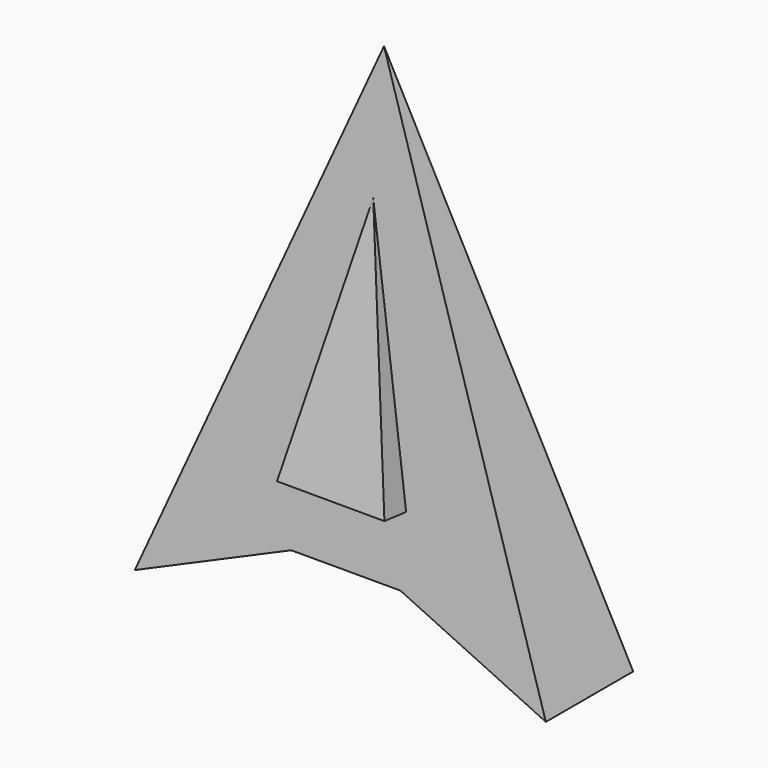
from build123d import *

# Parameters (mm, degrees)
F3_DEPTH  = 12.7
F5_DEPTH  = 67.0368353671
F6_DEPTH  = 28.5643014728
F8_DEPTH  = 6.35
F10_DEPTH = 64.56300866
F12_DEPTH = 6.35
F14_DEPTH = 65.6539037047


# Not quite as in the source:
# - the program builds the solid bodies; features that only make, move or delete a surface that nothing else refers to are left out


with BuildPart() as f3:
    # F2 (on Front) → F3 (new body, symmetric)
    with BuildSketch(Plane.XZ):
        Polygon((-28.5633014728, 34.2233732831), (6.5362669471, 49.0433023226), (31.9362669471, 49.0433023226), (67.0358353671, 34.2233732831), (19.2362669471, 151.884757173), align=None)
    extrude(amount=F3_DEPTH, both=True)

    # F4 (on Right) → F5 (cut, through all)
    with BuildSketch(Plane.YZ):
        Polygon((-12.7, 151.884757173), (-12.7, 49.0433023226), (-11.1003834344, 49.0433023226), (0, 151.884757173), align=None)
        Polygon((11.1003834344, 49.0433023226), (12.7, 49.0433023226), (12.7, 151.884757173), (0, 151.884757173), align=None)
        Polygon((-12.7, 49.0433023226), (-12.7, 34.2233732831), (-11.1003834344, 49.0433023226), align=None)
        Polygon((11.1003834344, 49.0433023226), (12.7, 34.2233732831), (12.7, 49.0433023226), align=None)
    extrude(amount=F5_DEPTH, mode=Mode.SUBTRACT)

    # F4 (on Right) → F6 (cut, through all)
    with BuildSketch(Plane.YZ):
        Polygon((-12.7, 151.884757173), (-12.7, 49.0433023226), (-11.1003834344, 49.0433023226), (0, 151.884757173), align=None)
        Polygon((11.1003834344, 49.0433023226), (12.7, 49.0433023226), (12.7, 151.884757173), (0, 151.884757173), align=None)
        Polygon((11.1003834344, 49.0433023226), (12.7, 34.2233732831), (12.7, 49.0433023226), align=None)
        Polygon((-12.7, 49.0433023226), (-12.7, 34.2233732831), (-11.1003834344, 49.0433023226), align=None)
    extrude(amount=-F6_DEPTH, mode=Mode.SUBTRACT)

    # F7 (on face) → F8 (join)
    with BuildSketch(Plane(origin=(0, 16.2051672418, 1.7491348237), x_dir=(-1, 0, 0), z_dir=(0, 0.9942252274, 0.1073135465))):
        Polygon((-6.5362669471, 60.7595853508), (-19.2362669471, 131.8038254976), (-31.9362669471, 60.7595853508), align=None)
    extrude(amount=F8_DEPTH)

    # F9 (on face) → F10 (cut, through all)
    with BuildSketch(Plane(origin=(-4.1912929855, -0.0804039557, 0.7449165901), x_dir=(0.0185928408, -0.9998216774, -0.0033044971), z_dir=(-0.9843951195, -0.0188842111, 0.1749560955))):
        Polygon((-15.6091843346, 67.4581627004), (-16.0814424902, 63.0134852894), (-2.1416171439, 134.1090394919), (-8.4560733481, 134.7799663477), align=None)
    extrude(amount=-F10_DEPTH, mode=Mode.SUBTRACT)

    # F11 (on face) → F12 (join)
    with BuildSketch(Plane(origin=(0, -16.2051672418, 1.7491348237), x_dir=(1, 0, 0), z_dir=(0, -0.9942252274, 0.1073135465))):
        Polygon((19.2987158189, 121.0772431274), (6.5362669471, 62.8382145463), (31.9300841439, 63.0873250248), align=None)
    extrude(amount=F12_DEPTH)

    # F13 (on face) → F14 (cut, through all)
    with BuildSketch(Plane(origin=(43.6030001695, 1.019222081, 9.442762247), x_dir=(-0.0223220606, 0.9997391444, -0.0048341149), z_dir=(0.9770893164, 0.0228395065, 0.2116006255))):
        Polygon((-16.230656346, 62.0519835601), (-16.7719699924, 56.9192946566), (-4.2322649759, 115.2756170682), (-10.5472424667, 115.9416195391), align=None)
    extrude(amount=-F14_DEPTH, mode=Mode.SUBTRACT)


solid = f3.part
